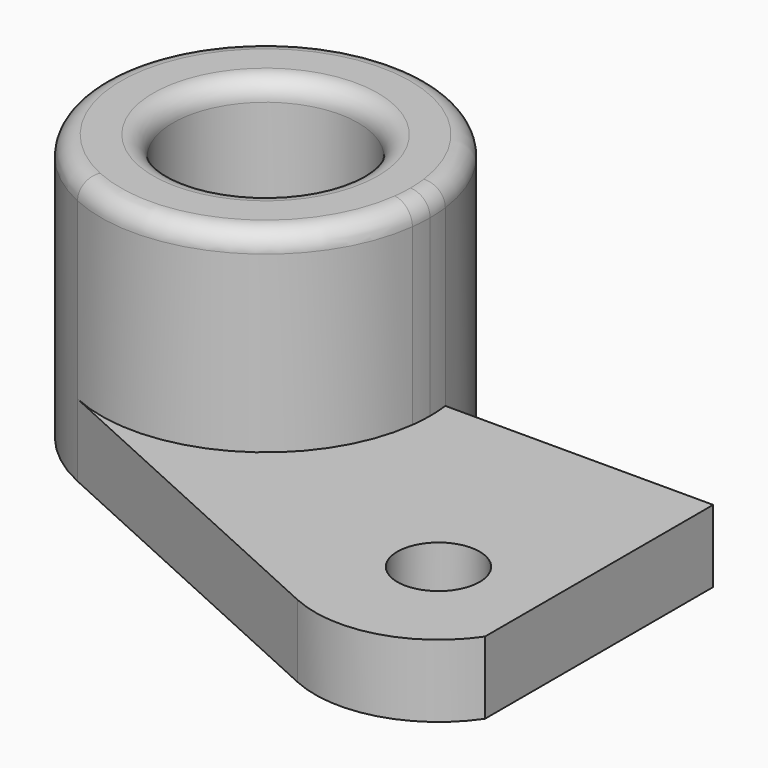
from build123d import *

# Parameters (mm, degrees)
F0_R     = 6.35
F1_DEPTH = 11.176
F0_R_2   = 16.256
F0_R_3   = 14.2875
F2_DEPTH = 41.148
F3_R     = 3.048
F4_R     = 3.048


with BuildPart() as f1:
    # F0 (on Top) → F1 (new body)
    with BuildSketch(Plane.XY):
        with BuildLine():
            ThreePointArc((-41.3472187621, 3.175), (-41.1978536154, 1.5906219786), (-41.148, 0))
            ThreePointArc((-41.148, 0), (-41.1978536154, -1.5906219786), (-41.3472187621, -3.175))
            Line((-41.3472187621, -3.175), (0, -3.175))
            Line((0, -3.175), (0, 0))
            Line((0, 0), (0, 3.175))
            Line((0, 3.175), (-41.3472187621, 3.175))
        make_face()
        with BuildLine():
            Line((0, -3.175), (-41.3472187621, -3.175))
            ThreePointArc((-41.3472187621, -3.175), (-54.1727312933, -22.1813598419), (-77.0827467531, -23.1123151339))
            Line((-77.0827467531, -23.1123151339), (-23.6490600649, -47.4677444402))
            ThreePointArc((-23.6490600649, -47.4677444402), (-10.6164287508, -48.4793380387), (0, -40.8527895955))
            Line((0, -40.8527895955), (0, -3.175))
        make_face()
        with Locations((-15.748, -30.1335080897)):
            Circle(F0_R, mode=Mode.SUBTRACT)
    extrude(amount=F1_DEPTH)

    # F0 (on Top) → F2 (join)
    with BuildSketch(Plane.XY):
        with BuildLine():
            ThreePointArc((-41.3472187621, -3.175), (-41.1978536154, -1.5906219786), (-41.148, 0))
            ThreePointArc((-41.148, 0), (-41.1978536154, 1.5906219786), (-41.3472187621, 3.175))
            ThreePointArc((-41.3472187621, 3.175), (-53.9498972239, 22.0555618029), (-76.6149503625, 23.3198737218))
            ThreePointArc((-76.6149503625, 23.3198737218), (-91.9467110203, 0.2558876856), (-77.0827467531, -23.1123151339))
            ThreePointArc((-77.0827467531, -23.1123151339), (-54.1727312933, -22.1813598419), (-41.3472187621, -3.175))
        make_face()
        with Locations((-66.548, 0)):
            Circle(F0_R_2, mode=Mode.SUBTRACT)
        with Locations((-66.548, 0)):
            Circle(F0_R_2)
        with Locations((-66.548, 0)):
            Circle(F0_R_3, mode=Mode.SUBTRACT)
    extrude(amount=F2_DEPTH)

    # F3
    f3_edges = [f1.edges().sort_by_distance(p)[0] for p in [
        (-91.748781, 3.175, 41.148),
    ]]
    fillet(f3_edges, radius=F3_R)

    # F4
    f4_edges = [f1.edges().sort_by_distance(p)[0] for p in [
        (-80.8355, 0, 41.148),
    ]]
    fillet(f4_edges, radius=F4_R)


solid = f1.part
